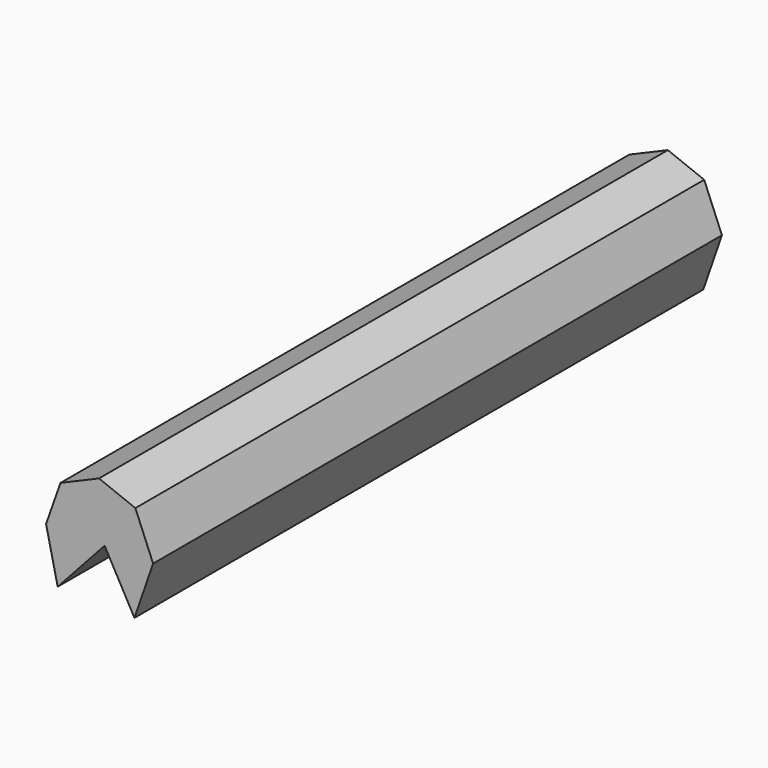
from build123d import *

# Parameters (mm, degrees)
F5_DEPTH = 508


# Not quite as in the source:
# - the program builds the solid bodies; features that only make, move or delete a surface that nothing else refers to are left out


with BuildPart() as f5:
    # F4 (on Front) → F5 (new body)
    with BuildSketch(Plane.XZ):
        Polygon((10.2848382667, 29.2012058198), (0, 0), (8.2863867283, -36.7476679385), (41.8159514666, 0), (63.1327554584, -38.524068892), (76.4557644725, 0), (63.7989118695, 30.7555589825), (37.8190502524, 40.969863534), align=None)
    extrude(amount=-F5_DEPTH)


solid = f5.part
